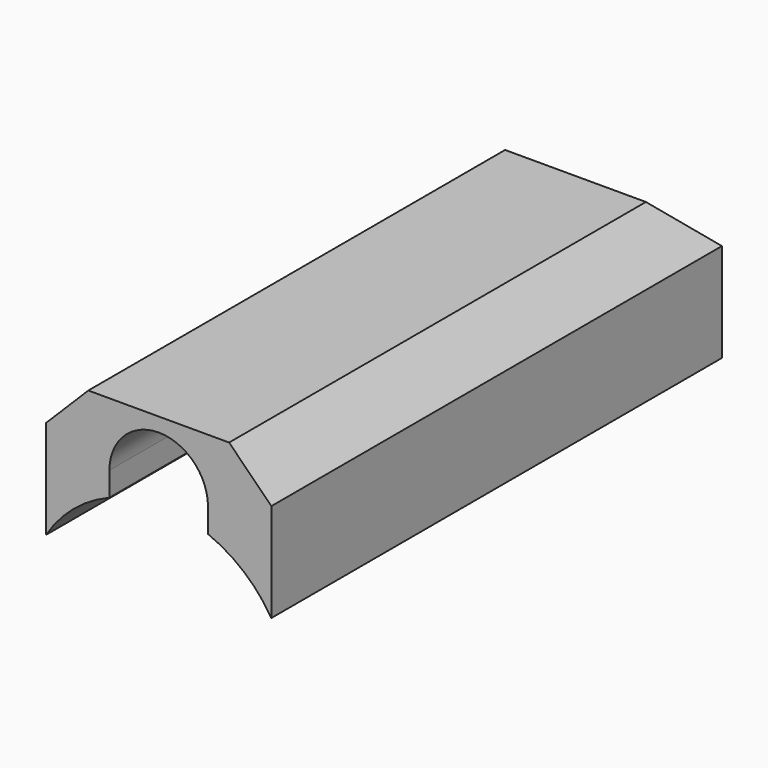
from build123d import *

# Parameters (mm, degrees)
F5_DEPTH  = 20
F6_SIZE   = 1.5
F7_SIZE   = 1.5
F11_DEPTH = 2.7510001


# Not quite as in the source:
# - a feature names something its author has since deleted; it is built from what else it names


with BuildPart() as f5:
    # F4 (on Front) → F5 (new body)
    with BuildSketch(Plane.XZ):
        with BuildLine():
            ThreePointArc((1.75, 4.3620522693), (3.0269919036, 3.5954582483), (4, 2.4677925359))
            Line((4, 2.4677925359), (4, 7.4677925359))
            Line((4, 7.4677925359), (-4, 7.4677925359))
            Line((-4, 7.4677925359), (-4, 2.4677925359))
            ThreePointArc((-4, 2.4677925359), (-3.0269919036, 3.5954582483), (-1.75, 4.3620522693))
            Line((-1.75, 4.3620522693), (-1.75, 5.2177925359))
            ThreePointArc((-1.75, 5.2177925359), (0, 6.9677925359), (1.75, 5.2177925359))
            Line((1.75, 5.2177925359), (1.75, 4.3620522693))
        make_face()
        with BuildLine():
            ThreePointArc((-1.75, 4.3620522693), (0, 4.7), (1.75, 4.3620522693))
            Line((1.75, 4.3620522693), (1.75, 5.2177925359))
            ThreePointArc((1.75, 5.2177925359), (0, 6.9677925359), (-1.75, 5.2177925359))
            Line((-1.75, 5.2177925359), (-1.75, 4.3620522693))
        make_face()
    extrude(amount=-F5_DEPTH)

    # F6
    f6_edges = [f5.edges().sort_by_distance(p)[0] for p in [
        (-4, 10, 7.467793),
        (4, 10, 7.467793),
    ]]
    chamfer(f6_edges, length=F6_SIZE)

    # F7
    f7_edges = [f5.edges().sort_by_distance(p)[0] for p in [
        (0, 20, 7.467793),
    ]]
    chamfer(f7_edges, length=F7_SIZE)

    # F9 (on offset) → F10 (revolve, cut)
    with BuildSketch(Plane.XY.offset(5.2177925359)):
        with BuildLine():
            Line((-1.75, 11.25), (-1.75, 0))
            Line((-1.75, 0), (0, 0))
            Line((0, 0), (0, 13))
            ThreePointArc((0, 13), (-1.2374368671, 12.4874368671), (-1.75, 11.25))
        make_face()
    revolve(axis=Axis((0, 6.5, 5.2177925359), (0, 1, 0)), mode=Mode.SUBTRACT)

    # F9 (on offset) → F11 (cut, through all)
    with BuildSketch(Plane.XY.offset(5.2177925359)):
        with BuildLine():
            Line((0, 13), (0, 0))
            Line((0, 0), (1.75, 0))
            Line((1.75, 0), (1.75, 11.25))
            ThreePointArc((1.75, 11.25), (1.2374368671, 12.4874368671), (0, 13))
        make_face()
        with BuildLine():
            Line((-1.75, 11.25), (-1.75, 0))
            Line((-1.75, 0), (0, 0))
            Line((0, 0), (0, 13))
            ThreePointArc((0, 13), (-1.2374368671, 12.4874368671), (-1.75, 11.25))
        make_face()
    extrude(amount=-F11_DEPTH, mode=Mode.SUBTRACT)


solid = f5.part
